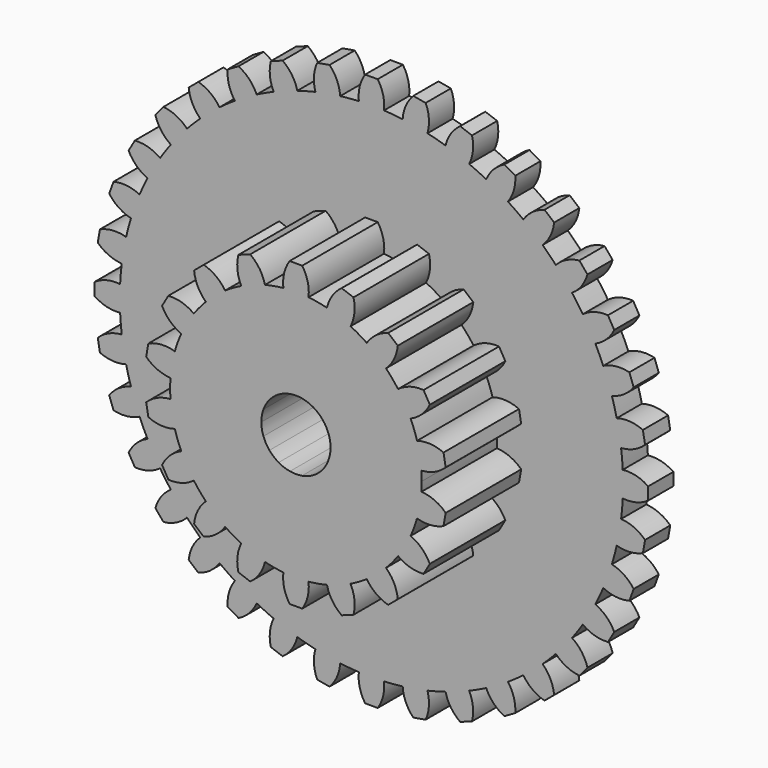
from build123d import *

# Parameters (mm, degrees)
F1_DEPTH = 2.5
F3_COUNT = 36
F2_R     = 5.5
F4_DEPTH = 25
F5_R     = 5.5
F6_DEPTH = 15
F7_COUNT = 18


with BuildPart() as f1:
    # F0 (on Front) → F1 (new body, symmetric)
    with BuildSketch(Plane.XZ):
        with BuildLine():
            ThreePointArc((-2, 39.9499687109), (-27.5680975042, -28.9827534924), (40, 0))
            ThreePointArc((40, 0), (28.9827534924, 27.5680975042), (2, 39.9499687109))
            ThreePointArc((2, 39.9499687109), (0, 40), (-2, 39.9499687109))
        make_face()
        with BuildLine():
            ThreePointArc((-2, 39.9499687109), (0, 40), (2, 39.9499687109))
            ThreePointArc((2, 39.9499687109), (1.8633168714, 42.0646915319), (1, 44))
            Line((1, 44), (-1, 44))
            ThreePointArc((-1, 44), (-1.8633168714, 42.0646915319), (-2, 39.9499687109))
        make_face()
    extrude(amount=F1_DEPTH, both=True)

    # F3: F1 ×36 about axis
    f3_axis = Axis((0, 0, 0), (0, -1, 0))


with BuildPart() as f1_1:
    add(f1.part)
    for i in range(1, F3_COUNT):
        add(f1.part.rotate(f3_axis, i * 360 / F3_COUNT))

    # F2 (on face) → F4 (cut)
    with BuildSketch(Plane.XZ.offset(2.5)):
        Circle(F2_R)
    extrude(amount=-F4_DEPTH, mode=Mode.SUBTRACT)



with BuildPart() as f6:
    # F5 (on face) → F6 (new body)
    with BuildSketch(Plane.XZ.offset(2.5)):
        with BuildLine():
            ThreePointArc((-2, 19.8997487421), (0, 20), (2, 19.8997487421))
            ThreePointArc((2, 19.8997487421), (1.8724139119, 22.0407014664), (1, 24))
            Line((1, 24), (-1, 24))
            ThreePointArc((-1, 24), (-1.8724139119, 22.0407014664), (-2, 19.8997487421))
        make_face()
        with BuildLine():
            ThreePointArc((-2, 19.8997487421), (-13.416407865, -14.8323969742), (20, 0))
            ThreePointArc((20, 0), (14.8323969742, 13.416407865), (2, 19.8997487421))
            ThreePointArc((2, 19.8997487421), (0, 20), (-2, 19.8997487421))
        make_face()
        Circle(F5_R, mode=Mode.SUBTRACT)
    extrude(amount=F6_DEPTH)


with BuildPart() as f1_2:
    add(f1_1.part)

    add(f6.part)  # F7 merges F6
    # F7: F6 ×18 about axis
    f7_axis = Axis((0, -2.5, 0), (0, 1, 0))
    for i in range(1, F7_COUNT):
        add(f6.part.rotate(f7_axis, i * 360 / F7_COUNT))


solid = f1_2.part
